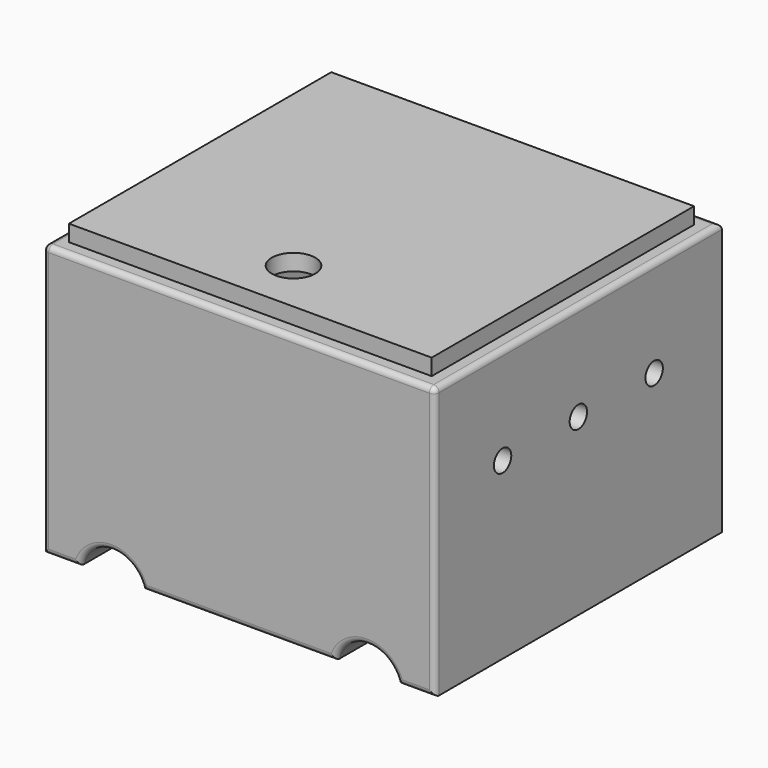
from build123d import *

# Parameters (mm, degrees)
F1_DEPTH      = 33
F0_R          = 1.6
F2_DEPTH      = 1.5
F3_R          = 2.35
F4_DEPTH      = 3
F5_R          = 1
F6_DEPTH      = 3
F8_DEPTH      = 21
F9_W          = 33.3554623196
F9_H          = 30.1534957824
F9_W_2        = 33.2154623196
F9_H_2        = 30.0134957824
F9_R          = 2
F10_DEPTH     = 1.5
F11_START     = -2
F11_DEPTH     = 1
F12_T4_ANGLE  = 198.8455092734
F12_T9_ANGLE  = 198.8455092734
F12_T11_DEPTH = 20.1905249807
F12_T13_DEPTH = 5.8452624903
F12_T15_DEPTH = 25.75
F12_T17_DEPTH = 5.8452624903
F12_T19_DEPTH = 35
F12_T21_DEPTH = 33.75
F12_T23_DEPTH = 38.5
F12_S27_W     = 0.51
F12_S27_H     = 0.51
F12_T28_DEPTH = 0.51
F12_S33_W     = 0.51
F12_S33_H     = 0.51
F12_T34_DEPTH = 0.51
F12_T42_ANGLE = 198.8455092734
F12_T44_ANGLE = 198.8455092734


# Not quite as in the source:
# - a fillet or chamfer that OpenCascade refuses, or shapes differently, is made with other operations: its cross-section is extruded or revolved along the edge and cut away or added


with BuildPart() as f1:
    # F0 (on Front) → F1 (new body)
    with BuildSketch(Plane.XZ):
        with BuildLine():
            Line((-21.2621615902, 57.3946547936), (-57.2621615902, 57.3946547936))
            Line((-57.2621615902, 57.3946547936), (-57.2621615902, 32.3946547936))
            Line((-57.2621615902, 32.3946547936), (-53.9168990998, 32.3946547936))
            ThreePointArc((-53.9168990998, 32.3946547936), (-51.0121615902, 34.6446547936), (-48.1074240805, 32.3946547936))
            Line((-48.1074240805, 32.3946547936), (-30.4168990998, 32.3946547936))
            ThreePointArc((-30.4168990998, 32.3946547936), (-27.5121615902, 34.6446547936), (-24.6074240805, 32.3946547936))
            Line((-24.6074240805, 32.3946547936), (-21.2621615902, 32.3946547936))
            Line((-21.2621615902, 32.3946547936), (-21.2621615902, 57.3946547936))
        make_face()
    extrude(amount=F1_DEPTH)

    # F0 (on Front) → F2 (join)
    with BuildSketch(Plane.XZ):
        with BuildLine():
            Line((-21.2621615902, 57.3946547936), (-57.2621615902, 57.3946547936))
            Line((-57.2621615902, 57.3946547936), (-57.2621615902, 32.3946547936))
            Line((-57.2621615902, 32.3946547936), (-53.9168990998, 32.3946547936))
            ThreePointArc((-53.9168990998, 32.3946547936), (-51.0121615902, 34.6446547936), (-48.1074240805, 32.3946547936))
            Line((-48.1074240805, 32.3946547936), (-30.4168990998, 32.3946547936))
            ThreePointArc((-30.4168990998, 32.3946547936), (-27.5121615902, 34.6446547936), (-24.6074240805, 32.3946547936))
            Line((-24.6074240805, 32.3946547936), (-21.2621615902, 32.3946547936))
            Line((-21.2621615902, 32.3946547936), (-21.2621615902, 57.3946547936))
        make_face()
        with BuildLine():
            ThreePointArc((-48.1074240805, 32.3946547936), (-51.0121615902, 34.6446547936), (-53.9168990998, 32.3946547936))
            ThreePointArc((-53.9168990998, 32.3946547936), (-51.0121615902, 28.6446547936), (-48.1074240805, 32.3946547936))
        make_face()
        with Locations((-51.0121615902, 31.6446547936)):
            Circle(F0_R, mode=Mode.SUBTRACT)
        with BuildLine():
            ThreePointArc((-30.4168990998, 32.3946547936), (-27.5121615902, 28.6446547936), (-24.6074240805, 32.3946547936))
            ThreePointArc((-24.6074240805, 32.3946547936), (-27.5121615902, 34.6446547936), (-30.4168990998, 32.3946547936))
        make_face()
        with Locations((-27.5121615902, 31.6446547936)):
            Circle(F0_R, mode=Mode.SUBTRACT)
    extrude(amount=F2_DEPTH)

    # F3 (on face) → F4 (cut)
    with BuildSketch(Plane(origin=(-57.2621615902, 0, 0), x_dir=(0, -1, 0), z_dir=(-1, 0, 0))):
        with Locations((10.5004208162, 49.5190024376)):
            Circle(F3_R)
        with Locations((22.4995791838, 49.5190024376)):
            Circle(F3_R)
    extrude(amount=-F4_DEPTH, mode=Mode.SUBTRACT)

    # F5 (on face) → F6 (cut)
    with BuildSketch(Plane.YZ.offset(-21.2621615902)):
        with Locations((-7.7914634645, 48.4387092292)):
            Circle(F5_R)
        with Locations((-16.5, 48.4387092292)):
            Circle(F5_R)
        with Locations((-25.2085365355, 48.4387092292)):
            Circle(F5_R)
    extrude(amount=-F6_DEPTH, mode=Mode.SUBTRACT)

    # F7 (on face) → F8 (cut)
    with BuildSketch(Plane.XY.offset(57.3946547936)):
        Polygon((-24.7621615902, -31.5), (-22.7621615902, -31.5), (-22.7621615902, -29.5), align=None)
        Polygon((-53.9776239097, -31.5), (-24.7621615902, -31.5), (-22.7621615902, -29.5), (-22.7621615902, -3.4865042176), (-24.7621615902, -1.4865042176), (-53.9776239097, -1.4865042176), (-55.9776239097, -3.4865042176), (-55.9776239097, -29.5), align=None)
        Polygon((-55.9776239097, -31.5), (-53.9776239097, -31.5), (-55.9776239097, -29.5), align=None)
        Polygon((-24.7621615902, -1.4865042176), (-22.7621615902, -3.4865042176), (-22.7621615902, -1.4865042176), align=None)
        Polygon((-55.9776239097, -1.4865042176), (-55.9776239097, -3.4865042176), (-53.9776239097, -1.4865042176), align=None)
    extrude(amount=-F8_DEPTH, mode=Mode.SUBTRACT)

    # F7 (on face) → F11 (join)
    with BuildSketch(Plane.XY.offset(57.3946547936).offset(F11_START)):
        Polygon((-24.7621615902, -31.5), (-22.7621615902, -31.5), (-22.7621615902, -29.5), align=None)
        Polygon((-55.9776239097, -31.5), (-53.9776239097, -31.5), (-55.9776239097, -29.5), align=None)
        Polygon((-24.7621615902, -1.4865042176), (-22.7621615902, -3.4865042176), (-22.7621615902, -1.4865042176), align=None)
        Polygon((-55.9776239097, -1.4865042176), (-55.9776239097, -3.4865042176), (-53.9776239097, -1.4865042176), align=None)
    extrude(amount=-F11_DEPTH)

    # F12: fillet of radius 0.5 on 15 edges, made by hand


with BuildPart() as f10:
    # F9 (on face) → F10 (new body)
    with BuildSketch(Plane.XY.offset(57.3946547936)):
        with Locations((-39.3698927499, -16.4932521088)):
            Rectangle(F9_W, F9_H)
        with Locations((-39.3698927499, -16.4932521088)):
            Rectangle(F9_W_2, F9_H_2, mode=Mode.SUBTRACT)
        with Locations((-39.3698927499, -16.4932521088)):
            Rectangle(F9_W_2, F9_H_2)
        with Locations((-39.3698927499, -26.6023594886)):
            Circle(F9_R, mode=Mode.SUBTRACT)
    extrude(amount=F10_DEPTH)


with BuildPart() as f12_tool2:
    # F12_s3 → F12_t4 (revolve)
    with BuildSketch(Plane(origin=(-6.4781934327, 0, 39.0353776982), x_dir=(0, 1, 0), z_dir=(0.1637177599, 0, -0.98650722))):
        with BuildLine():
            ThreePointArc((-2, -48.1430737202), (-1.6464466094, -47.9966271108), (-1.5, -47.6430737202))
            Line((-1.5, -47.6430737202), (-1.5, -48.1430737202))
            Line((-1.5, -48.1430737202), (-2, -48.1430737202))
        make_face()
    revolve(axis=Axis((-51.0121615902, -1.5, 31.6446547936), (0, 1, 0)), revolution_arc=F12_T4_ANGLE)

    split(bisect_by=Plane.XY.offset(32.3946547936), keep=Keep.TOP)


with BuildPart() as f1_1:
    add(f1.part)

    # F12_t1: union F12_tool2
    add(f12_tool2.part)


with BuildPart() as f12_tool7:
    # F12_s8 → F12_t9 (revolve)
    with BuildSketch(Plane(origin=(-5.8483110673, 0, 35.2399220219), x_dir=(0, 1, 0), z_dir=(0.1637177599, 0, -0.98650722))):
        with BuildLine():
            ThreePointArc((-2, -24.9601540504), (-1.6464466094, -24.813707441), (-1.5, -24.4601540504))
            Line((-1.5, -24.4601540504), (-1.5, -24.9601540504))
            Line((-1.5, -24.9601540504), (-2, -24.9601540504))
        make_face()
    revolve(axis=Axis((-27.5121615902, -1.5, 31.6446547936), (0, 1, 0)), revolution_arc=F12_T9_ANGLE)

    split(bisect_by=Plane.XY.offset(32.3946547936), keep=Keep.TOP)


with BuildPart() as f1_2:
    add(f1_1.part)

    # F12_t6: union F12_tool7
    add(f12_tool7.part)

    # F12_s12 → F12_t11 (cut)
    with BuildSketch(Plane.YZ.offset(-49.3574240805)):
        with BuildLine():
            ThreePointArc((-33, 32.8946547936), (-32.8535533906, 32.541101403), (-32.5, 32.3946547936))
            Line((-32.5, 32.3946547936), (-33, 32.3946547936))
            Line((-33, 32.3946547936), (-33, 32.8946547936))
        make_face()
    extrude(amount=F12_T11_DEPTH, mode=Mode.SUBTRACT)

    # F12_s14 → F12_t13 (cut)
    with BuildSketch(Plane.YZ.offset(-25.8574240805)):
        with BuildLine():
            ThreePointArc((-33, 32.8946547936), (-32.8535533906, 32.541101403), (-32.5, 32.3946547936))
            Line((-32.5, 32.3946547936), (-33, 32.3946547936))
            Line((-33, 32.3946547936), (-33, 32.8946547936))
        make_face()
    extrude(amount=F12_T13_DEPTH, mode=Mode.SUBTRACT)

    # F12_s16 → F12_t15 (cut)
    with BuildSketch(Plane.XY.offset(31.1446547936)):
        with BuildLine():
            ThreePointArc((-21.2621615902, -32.5), (-21.4086081996, -32.8535533906), (-21.7621615902, -33))
            Line((-21.7621615902, -33), (-21.2621615902, -33))
            Line((-21.2621615902, -33), (-21.2621615902, -32.5))
        make_face()
        with BuildLine():
            ThreePointArc((-57.2621615902, -32.5), (-57.1157149808, -32.8535533906), (-56.7621615902, -33))
            Line((-56.7621615902, -33), (-57.2621615902, -33))
            Line((-57.2621615902, -33), (-57.2621615902, -32.5))
        make_face()
    extrude(amount=F12_T15_DEPTH, mode=Mode.SUBTRACT)

    # F12_s18 → F12_t17 (cut)
    with BuildSketch(Plane.YZ.offset(-58.5121615902)):
        with BuildLine():
            ThreePointArc((-33, 32.8946547936), (-32.8535533906, 32.541101403), (-32.5, 32.3946547936))
            Line((-32.5, 32.3946547936), (-33, 32.3946547936))
            Line((-33, 32.3946547936), (-33, 32.8946547936))
        make_face()
    extrude(amount=F12_T17_DEPTH, mode=Mode.SUBTRACT)

    # F12_s20 → F12_t19 (cut)
    with BuildSketch(Plane.YZ.offset(-56.7621615902)):
        with BuildLine():
            ThreePointArc((-32.5, 57.3946547936), (-32.8535533906, 57.2482081841), (-33, 56.8946547936))
            Line((-33, 56.8946547936), (-33, 57.3946547936))
            Line((-33, 57.3946547936), (-32.5, 57.3946547936))
        make_face()
    extrude(amount=F12_T19_DEPTH, mode=Mode.SUBTRACT)

    # F12_s22 → F12_t21 (cut)
    with BuildSketch(Plane.XZ.offset(-1.25)):
        with BuildLine():
            ThreePointArc((-56.7621615902, 57.3946547936), (-57.1157149808, 57.2482081841), (-57.2621615902, 56.8946547936))
            Line((-57.2621615902, 56.8946547936), (-57.2621615902, 57.3946547936))
            Line((-57.2621615902, 57.3946547936), (-56.7621615902, 57.3946547936))
        make_face()
        with BuildLine():
            ThreePointArc((-21.7621615902, 57.3946547936), (-21.4086081996, 57.2482081841), (-21.2621615902, 56.8946547936))
            Line((-21.2621615902, 56.8946547936), (-21.2621615902, 57.3946547936))
            Line((-21.2621615902, 57.3946547936), (-21.7621615902, 57.3946547936))
        make_face()
    extrude(amount=F12_T21_DEPTH, mode=Mode.SUBTRACT)

    # F12_s24 → F12_t23 (cut)
    with BuildSketch(Plane.YZ.offset(-58.5121615902)):
        with BuildLine():
            ThreePointArc((-0.5, 57.3946547936), (-0.1464466094, 57.2482081841), (0, 56.8946547936))
            Line((0, 56.8946547936), (0, 57.3946547936))
            Line((0, 57.3946547936), (-0.5, 57.3946547936))
        make_face()
    extrude(amount=F12_T23_DEPTH, mode=Mode.SUBTRACT)


with BuildPart() as f12_tool26:
    # F12_s27 → F12_t28 (new body)
    with BuildSketch(Plane.XY.offset(56.8946547936)):
        with Locations((-21.5071615902, -32.755)):
            Rectangle(F12_S27_W, F12_S27_H)
    extrude(amount=F12_T28_DEPTH)

    # F12_s29 → F12_t30 (revolve, cut)
    with BuildSketch(Plane(origin=(-21.7621615902, -32.5, 56.8946547936), x_dir=(-0.7071067812, 0.7071067812, 0), z_dir=(0.7071067812, 0.7071067812, 0))):
        with BuildLine():
            ThreePointArc((0, -0.5), (0.5, 0), (0, 0.5))
            Line((0, 0.5), (0, -0.5))
        make_face()
    revolve(axis=Axis((-21.7621615902, -32.5, 56.8946547936), (0, 0, 1)), mode=Mode.SUBTRACT)


with BuildPart() as f1_3:
    add(f1_2.part)

    # F12_t25: cut F12_tool26
    add(f12_tool26.part, mode=Mode.SUBTRACT)


with BuildPart() as f12_tool32:
    # F12_s33 → F12_t34 (new body)
    with BuildSketch(Plane.XY.offset(56.8946547936)):
        with Locations((-57.0171615902, -32.755)):
            Rectangle(F12_S33_W, F12_S33_H)
    extrude(amount=F12_T34_DEPTH)

    # F12_s35 → F12_t36 (revolve, cut)
    with BuildSketch(Plane(origin=(-56.7621615902, -32.5, 56.8946547936), x_dir=(0.7071067812, 0.7071067812, 0), z_dir=(0.7071067812, -0.7071067812, 0))):
        with BuildLine():
            ThreePointArc((0, -0.5), (0.5, 0), (0, 0.5))
            Line((0, 0.5), (0, -0.5))
        make_face()
    revolve(axis=Axis((-56.7621615902, -32.5, 56.8946547936), (0, 0, 1)), mode=Mode.SUBTRACT)


with BuildPart() as f1_4:
    add(f1_3.part)

    # F12_t31: cut F12_tool32
    add(f12_tool32.part, mode=Mode.SUBTRACT)

    # F12_s37 → F12_t38 (revolve, cut)
    with BuildSketch(Plane.XY.offset(31.6446547936)):
        with BuildLine():
            ThreePointArc((-25.9121615902, -1), (-25.7657149808, -1.3535533906), (-25.4121615902, -1.5))
            Line((-25.4121615902, -1.5), (-25.9121615902, -1.5))
            Line((-25.9121615902, -1.5), (-25.9121615902, -1))
        make_face()
    revolve(axis=Axis((-27.5121615902, -1.5, 31.6446547936), (0, -1, 0)), mode=Mode.SUBTRACT)

    # F12_s39 → F12_t40 (revolve, cut)
    with BuildSketch(Plane.XY.offset(31.6446547936)):
        with BuildLine():
            ThreePointArc((-49.4121615902, -1), (-49.2657149808, -1.3535533906), (-48.9121615902, -1.5))
            Line((-48.9121615902, -1.5), (-49.4121615902, -1.5))
            Line((-49.4121615902, -1.5), (-49.4121615902, -1))
        make_face()
    revolve(axis=Axis((-51.0121615902, -1.5, 31.6446547936), (0, -1, 0)), mode=Mode.SUBTRACT)

    # F12_s41 → F12_t42 (revolve, cut)
    with BuildSketch(Plane(origin=(-6.4781934327, 0, 39.0353776982), x_dir=(0, 1, 0), z_dir=(0.1637177599, 0, -0.98650722))):
        with BuildLine():
            ThreePointArc((-33, -48.6430737202), (-32.8535533906, -48.2895203296), (-32.5, -48.1430737202))
            Line((-32.5, -48.1430737202), (-33, -48.1430737202))
            Line((-33, -48.1430737202), (-33, -48.6430737202))
        make_face()
    revolve(axis=Axis((-51.0121615902, -33, 31.6446547936), (0, 1, 0)), revolution_arc=F12_T42_ANGLE, mode=Mode.SUBTRACT)

    # F12_s43 → F12_t44 (revolve, cut)
    with BuildSketch(Plane(origin=(-5.8483110673, 0, 35.2399220219), x_dir=(0, 1, 0), z_dir=(0.1637177599, 0, -0.98650722))):
        with BuildLine():
            ThreePointArc((-33, -25.4601540504), (-32.8535533906, -25.1066006599), (-32.5, -24.9601540504))
            Line((-32.5, -24.9601540504), (-33, -24.9601540504))
            Line((-33, -24.9601540504), (-33, -25.4601540504))
        make_face()
    revolve(axis=Axis((-27.5121615902, -33, 31.6446547936), (0, 1, 0)), revolution_arc=F12_T44_ANGLE, mode=Mode.SUBTRACT)


solid = Compound([f10.part, f1_4.part])
